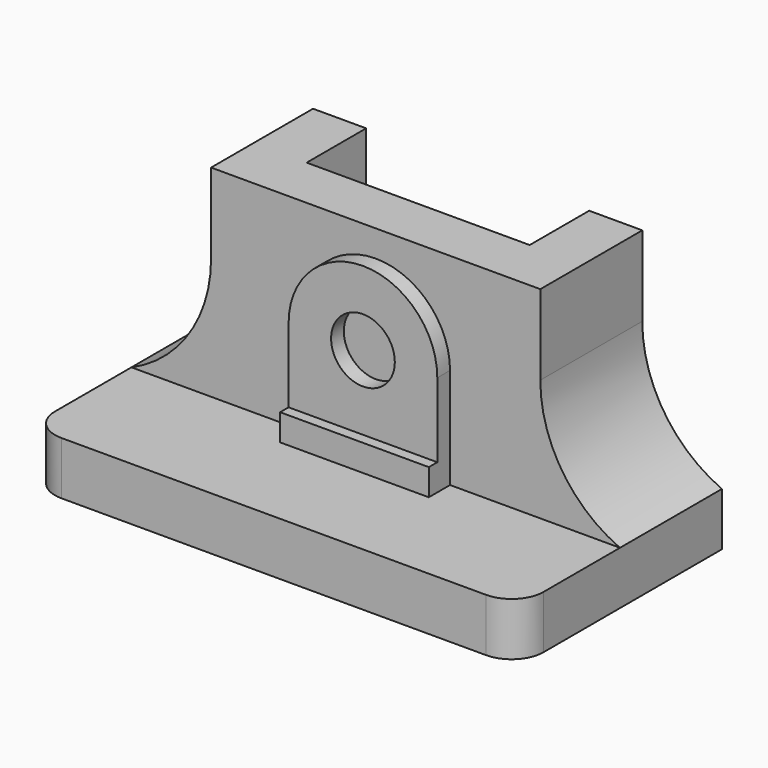
from build123d import *

# Parameters (mm, degrees)
F1_DEPTH    = 48
F0_W        = 42
F0_H        = 14
F2_DEPTH    = 10
F3_T1_DEPTH = 24
F4_T1_DEPTH = 24
F5_R        = 6
F6_DEPTH    = 3
F5_W        = 28
F5_H        = 5
F7_DEPTH    = 3
F8_R        = 6
F9_R        = 6
F10_W       = 28
F10_H       = 5
F11_DEPTH   = 5


# Not quite as in the source:
# - a fillet or chamfer that OpenCascade refuses, or shapes differently, is made with other operations: its cross-section is extruded or revolved along the edge and cut away or added


with BuildPart() as f1:
    # F0 (on Top) → F1 (new body)
    with BuildSketch(Plane.XY):
        Polygon((31, 0), (31, 24), (21, 24), (21, 10), (-21, 10), (-21, 24), (-31, 24), (-31, 0), align=None)
    extrude(amount=F1_DEPTH)

    # F0 (on Top) → F2 (join)
    with BuildSketch(Plane.XY):
        Polygon((-46, -24), (46, -24), (46, 24), (31, 24), (31, 0), (-31, 0), (-31, 24), (-46, 24), align=None)
        Polygon((31, 0), (31, 24), (21, 24), (21, 10), (-21, 10), (-21, 24), (-31, 24), (-31, 0), align=None)
        with Locations((0, 17)):
            Rectangle(F0_W, F0_H)
    extrude(amount=F2_DEPTH)

    # F3: fillet of radius 25 on 1 edges, made by hand

    # F3_s2 → F3_t1 (join)
    with BuildSketch(Plane.XZ.offset(-24)):
        with BuildLine():
            ThreePointArc((46, 10), (35.0834993366, 19.2198145372), (31, 32.9128784748))
            Line((31, 32.9128784748), (31, 10))
            Line((31, 10), (46, 10))
        make_face()
    extrude(amount=F3_T1_DEPTH)

    # F4: fillet of radius 25 on 1 edges, made by hand

    # F4_s2 → F4_t1 (join)
    with BuildSketch(Plane.XZ.offset(-24)):
        with BuildLine():
            ThreePointArc((-31, 32.9128784748), (-35.0834993366, 19.2198145372), (-46, 10))
            Line((-46, 10), (-31, 10))
            Line((-31, 10), (-31, 32.9128784748))
        make_face()
    extrude(amount=F4_T1_DEPTH)

    # F5 (on face) → F6 (join)
    with BuildSketch(Plane.XZ):
        with BuildLine():
            Line((14, 15), (14, 29))
            ThreePointArc((14, 29), (0, 43), (-14, 29))
            Line((-14, 29), (-14, 15))
            Line((-14, 15), (14, 15))
        make_face()
        with Locations((0, 29)):
            Circle(F5_R, mode=Mode.SUBTRACT)
    extrude(amount=F6_DEPTH)

    # F5 (on face) → F7 (join)
    with BuildSketch(Plane.XZ):
        with BuildLine():
            Line((14, 15), (14, 29))
            ThreePointArc((14, 29), (0, 43), (-14, 29))
            Line((-14, 29), (-14, 15))
            Line((-14, 15), (14, 15))
        make_face()
        with Locations((0, 29)):
            Circle(F5_R, mode=Mode.SUBTRACT)
        with Locations((0, 12.5)):
            Rectangle(F5_W, F5_H)
    extrude(amount=F7_DEPTH)

    # F8
    f8_edges = [f1.edges().sort_by_distance(p)[0] for p in [
        (46, -24, 5),
    ]]
    fillet(f8_edges, radius=F8_R)

    # F9
    f9_edges = [f1.edges().sort_by_distance(p)[0] for p in [
        (-46, -24, 5),
    ]]
    fillet(f9_edges, radius=F9_R)

    # F10 (on face) → F11 (join)
    with BuildSketch(Plane.XZ):
        with Locations((0, 12.5)):
            Rectangle(F10_W, F10_H)
    extrude(amount=F11_DEPTH)


solid = f1.part
